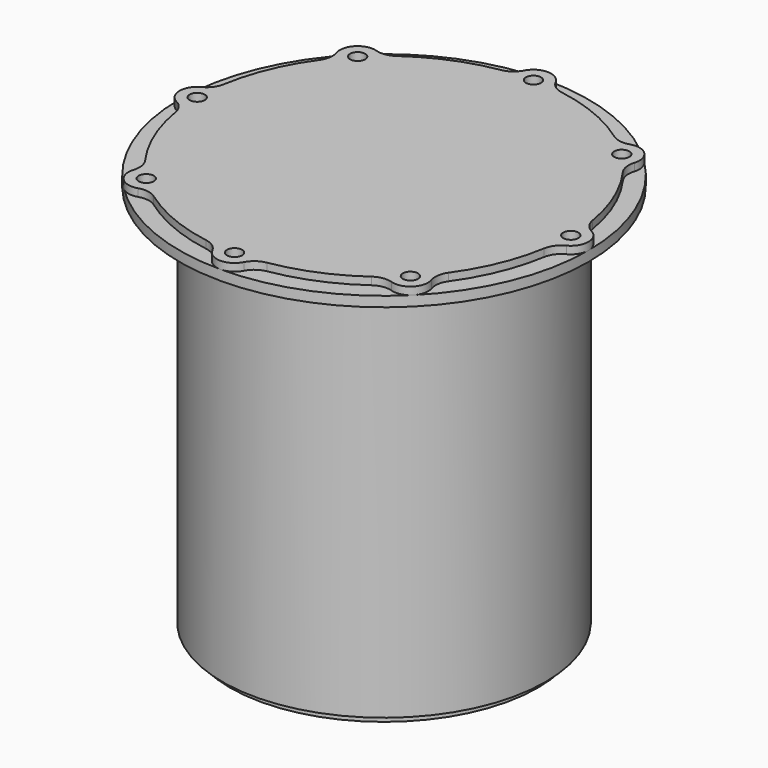
from build123d import *

# Parameters (mm, degrees)
F0_R     = 101.6
F0_R_2   = 96.8248
F1_DEPTH = 241.3
F2_R     = 96.266
F2_R_2   = 82.55
F3_DEPTH = 4.7752
F4_R     = 128.5875
F4_R_2   = 4.7625
F4_R_3   = 103.1875
F5_DEPTH = 6.35
F7_R     = 96.8248
F8_DEPTH = 4.7752
F6_R     = 4.7625
F9_DEPTH = 4.7752
F10_R    = 12.7


with BuildPart() as f1:
    # F0 (on Top) → F1 (new body)
    with BuildSketch(Plane.XY):
        Circle(F0_R)
        Circle(F0_R_2, mode=Mode.SUBTRACT)
    extrude(amount=F1_DEPTH)


with BuildPart() as f3:
    # F2 (on Top) → F3 (new body)
    with BuildSketch(Plane.XY):
        Circle(F2_R)
        Circle(F2_R_2, mode=Mode.SUBTRACT)
    extrude(amount=F3_DEPTH)


with BuildPart() as f5:
    # F4 (on face) → F5 (new body)
    with BuildSketch(Plane.XY.offset(241.3)):
        Circle(F4_R)
        with Locations((-83.0673691199, -83.0673691199)):
            Circle(F4_R_2, mode=Mode.SUBTRACT)
        with Locations((0, -117.475)):
            Circle(F4_R_2, mode=Mode.SUBTRACT)
        with Locations((83.0673691199, -83.0673691199)):
            Circle(F4_R_2, mode=Mode.SUBTRACT)
        with Locations((-117.475, 0)):
            Circle(F4_R_2, mode=Mode.SUBTRACT)
        with Locations((-83.0673691199, 83.0673691199)):
            Circle(F4_R_2, mode=Mode.SUBTRACT)
        Circle(F4_R_3, mode=Mode.SUBTRACT)
        with Locations((117.475, 0)):
            Circle(F4_R_2, mode=Mode.SUBTRACT)
        with Locations((0, 117.475)):
            Circle(F4_R_2, mode=Mode.SUBTRACT)
        with Locations((83.0673691199, 83.0673691199)):
            Circle(F4_R_2, mode=Mode.SUBTRACT)
    extrude(amount=F5_DEPTH)


with BuildPart() as f8:
    # F7 (on face) → F8 (new body)
    with BuildSketch(Plane(origin=(0, 0, 0), x_dir=(1, 0, 0), z_dir=(0, 0, -1))):
        Circle(F7_R)
    extrude(amount=F8_DEPTH)


with BuildPart() as f9:
    # F6 (on face) → F9 (new body)
    with BuildSketch(Plane.XY.offset(247.65)):
        with BuildLine():
            ThreePointArc((74.8369897921, 90.5527502832), (44.9557362171, 108.5327480818), (11.1127208148, 116.9482067459))
            ThreePointArc((11.1127208148, 116.9482067459), (0, 128.6002), (-11.1127208148, 116.9482067459))
            ThreePointArc((-11.1127208148, 116.9482067459), (-44.9557362171, 108.5327480818), (-74.8369897921, 90.5527502832))
            ThreePointArc((-74.8369897921, 90.5527502832), (-90.9340734819, 90.9340734819), (-90.5527502832, 74.8369897921))
            ThreePointArc((-90.5527502832, 74.8369897921), (-108.5327480818, 44.9557362171), (-116.9482067459, 11.1127208148))
            ThreePointArc((-116.9482067459, 11.1127208148), (-128.6002, 0), (-116.9482067459, -11.1127208148))
            ThreePointArc((-116.9482067459, -11.1127208148), (-108.5327480818, -44.9557362171), (-90.5527502832, -74.8369897921))
            ThreePointArc((-90.5527502832, -74.8369897921), (-90.9340734819, -90.9340734819), (-74.8369897921, -90.5527502832))
            ThreePointArc((-74.8369897921, -90.5527502832), (-44.9557362171, -108.5327480818), (-11.1127208148, -116.9482067459))
            ThreePointArc((-11.1127208148, -116.9482067459), (0, -128.6002), (11.1127208148, -116.9482067459))
            ThreePointArc((11.1127208148, -116.9482067459), (44.9557362171, -108.5327480818), (74.8369897921, -90.5527502832))
            ThreePointArc((74.8369897921, -90.5527502832), (90.9340734819, -90.9340734819), (90.5527502832, -74.8369897921))
            ThreePointArc((90.5527502832, -74.8369897921), (108.5327480818, -44.9557362171), (116.9482067459, -11.1127208148))
            ThreePointArc((116.9482067459, -11.1127208148), (128.6002, 0), (116.9482067459, 11.1127208148))
            ThreePointArc((116.9482067459, 11.1127208148), (108.5327480818, 44.9557362171), (90.5527502832, 74.8369897921))
            ThreePointArc((90.5527502832, 74.8369897921), (90.9340734819, 90.9340734819), (74.8369897921, 90.5527502832))
        make_face()
        with Locations((-83.0673691199, -83.0673691199)):
            Circle(F6_R, mode=Mode.SUBTRACT)
        with Locations((0, -117.475)):
            Circle(F6_R, mode=Mode.SUBTRACT)
        with Locations((83.0673691199, -83.0673691199)):
            Circle(F6_R, mode=Mode.SUBTRACT)
        with Locations((-117.475, 0)):
            Circle(F6_R, mode=Mode.SUBTRACT)
        with Locations((-83.0673691199, 83.0673691199)):
            Circle(F6_R, mode=Mode.SUBTRACT)
        with Locations((117.475, 0)):
            Circle(F6_R, mode=Mode.SUBTRACT)
        with Locations((0, 117.475)):
            Circle(F6_R, mode=Mode.SUBTRACT)
        with Locations((83.0673691199, 83.0673691199)):
            Circle(F6_R, mode=Mode.SUBTRACT)
    extrude(amount=F9_DEPTH)

    # F10
    f10_edges = [f9.edges().sort_by_distance(p)[0] for p in [
        (74.83699, 90.55275, 250.0376),
        (90.55275, 74.83699, 250.0376),
        (11.112721, 116.948207, 250.0376),
        (-11.112721, 116.948207, 250.0376),
        (-74.83699, 90.55275, 250.0376),
        (-90.55275, 74.83699, 250.0376),
        (-116.948207, 11.112721, 250.0376),
        (-116.948207, -11.112721, 250.0376),
        (-90.55275, -74.83699, 250.0376),
        (-74.83699, -90.55275, 250.0376),
        (-11.112721, -116.948207, 250.0376),
        (74.83699, -90.55275, 250.0376),
        (90.55275, -74.83699, 250.0376),
        (116.948207, 11.112721, 250.0376),
        (116.948207, -11.112721, 250.0376),
        (11.112721, -116.948207, 250.0376),
    ]]
    fillet(f10_edges, radius=F10_R)


solid = Compound([f1.part, f3.part, f5.part, f8.part, f9.part])
